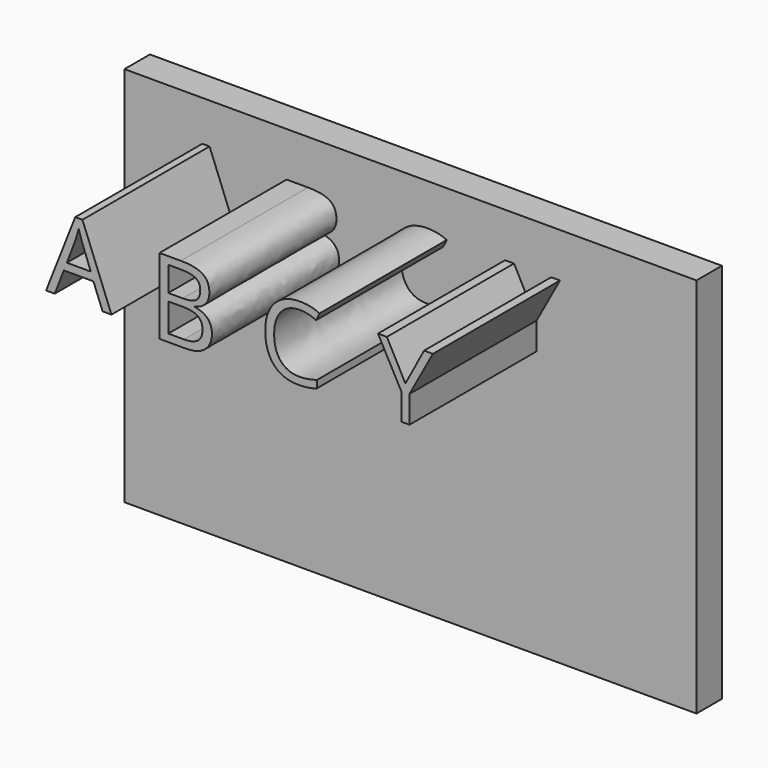
from build123d import *

# Parameters (mm, degrees)
F0_W           = 90
F0_H           = 60
F1_DEPTH       = 5
F2_TEXT_SIZE   = 16.2563739448
F2_TEXT_SIZE_2 = 16.6732080591
F2_TEXT_SIZE_3 = 15.8395450045
F2_TEXT_SIZE_4 = 15.4227160642
F3_DEPTH       = 25


# Not quite as in the source:
# - Text() gives the source's letters only with a copy of the font that has no kerning and outlines rounded to 1/6400 em; it was checked with that copy


with BuildPart() as f1:
    # F0 (on Front) → F1 (new body)
    with BuildSketch(Plane.XZ):
        with Locations((3.8241893053, 3.6314051988)):
            Rectangle(F0_W, F0_H)
    extrude(amount=F1_DEPTH)

    # F2 (on face) → F3 (join)
    with BuildSketch(Plane.XZ.offset(5)):
        with Locations((-33.5126891732, 15.6227750704)):
            Text('A', F2_TEXT_SIZE, font='Open Sans', text_align=(TextAlign.LEFT, TextAlign.BOTTOM))
        with Locations((-17.3063315451, 14.722420834)):
            Text('B', F2_TEXT_SIZE_2, font='Open Sans', text_align=(TextAlign.LEFT, TextAlign.BOTTOM))
        with Locations((0, 15.6227750704)):
            Text('C', F2_TEXT_SIZE_3, font='Open Sans', text_align=(TextAlign.LEFT, TextAlign.BOTTOM))
        with Locations((18.7077894807, 15.6227750704)):
            Text('Y', F2_TEXT_SIZE_4, font='Open Sans', text_align=(TextAlign.LEFT, TextAlign.BOTTOM))
    extrude(amount=F3_DEPTH)


solid = f1.part
